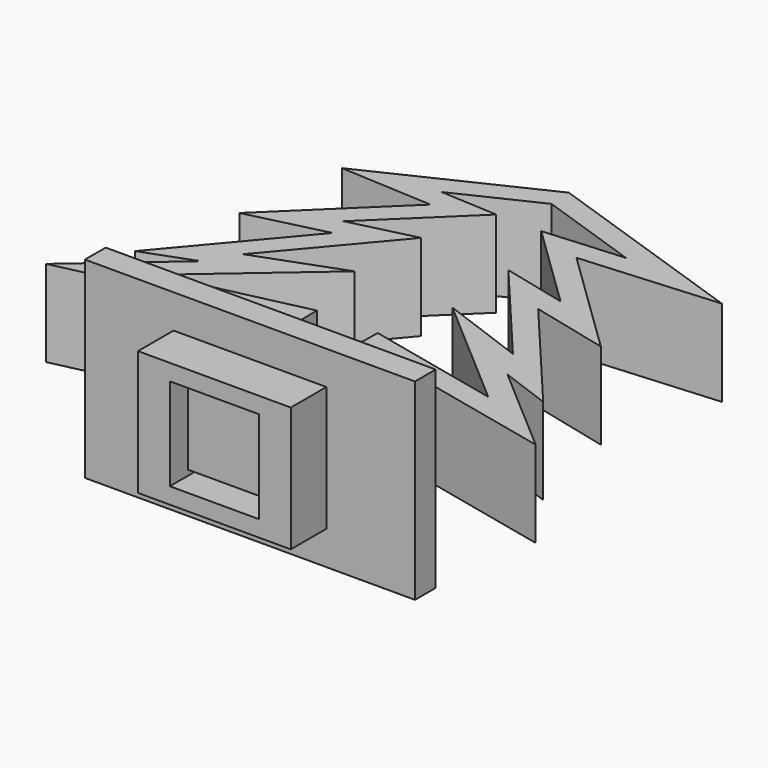
from build123d import *

# Parameters (mm, degrees)
F1_DEPTH = 25.4
F2_W     = 96.9438627362
F2_H     = 56.4742647111
F2_W_2   = 44.8701865971
F2_H_2   = 36.6715993732
F2_W_3   = 26.1676702648
F2_H_3   = 27.1369842812
F3_DEPTH = 7.62
F4_DEPTH = 13.05744


with BuildPart() as f1:
    # F0 (on Top) → F1 (new body)
    with BuildSketch(Plane.XY):
        Polygon((-15.2002724628, -7.9219630817), (-14.8288337448, -42.0940224084), (0, -42.0940224084), (14.8288337448, -42.0940224084), (15.2002724628, -7.9219630817), (71.9137688096, -20.7102910067), (45.0371085278, 2.5013713437), (59.9321083919, -2.9983216828), (30.2034030994, 32.3314461975), (53.0932784976, 26.7257584044), (21.1701166571, 57.6666764014), (61.4833603316, 60.6945607437), (-0.3977347554, 81.830812644), (-48.6371593785, 58.8133267539), (-21.4750114589, 57.3711629086), (-53.0932784976, 26.7257584044), (-30.2034030994, 32.3314461975), (-59.9321083919, -2.9983216828), (-45.0371085278, 2.5013713437), (-71.9137688096, -20.7102910067), align=None)
        Polygon((8.5474811494, -35.744022578), (0, -35.744022578), (-8.5474811494, -35.744022578), (-8.9360065758, 0), (-48.5652536154, -8.9360000566), (-14.3753122538, 20.5916780978), (-39.6292470396, 11.267147027), (-12.8212254494, 43.1259572506), (-31.858805567, 38.4636893868), (-6.6048740409, 62.940582633), (-23.3757123351, 63.8310238719), (0, 74.9847665429), (30.0963129848, 64.7049993277), (6.6048740409, 62.940582633), (31.858805567, 38.4636893868), (12.8212254494, 43.1259572506), (39.6292470396, 11.267147027), (14.3753122538, 20.5916780978), (48.5652536154, -8.9360000566), (8.9360065758, 0), align=None, mode=Mode.SUBTRACT)
    extrude(amount=F1_DEPTH)


with BuildPart() as f3:
    # F2 (on face) → F3 (new body)
    with BuildSketch(Plane(origin=(0, -35.744022578, 0), x_dir=(-1, 0, 0), z_dir=(0, 1, 0))):
        with Locations((0, 12.0169725269)):
            Rectangle(F2_W, F2_H)
        with Locations((0, 12.0169725269)):
            Rectangle(F2_W_2, F2_H_2, mode=Mode.SUBTRACT)
        with Locations((0, 12.0169725269)):
            Rectangle(F2_W_2, F2_H_2)
        with Locations((0, 12.0169725269)):
            Rectangle(F2_W_3, F2_H_3, mode=Mode.SUBTRACT)
    extrude(amount=F3_DEPTH)

    # F2 (on face) → F4 (join)
    with BuildSketch(Plane(origin=(0, -35.744022578, 0), x_dir=(-1, 0, 0), z_dir=(0, 1, 0))):
        with Locations((0, 12.0169725269)):
            Rectangle(F2_W_2, F2_H_2)
        with Locations((0, 12.0169725269)):
            Rectangle(F2_W_3, F2_H_3, mode=Mode.SUBTRACT)
    extrude(amount=-F4_DEPTH)


solid = Compound([f1.part, f3.part])
